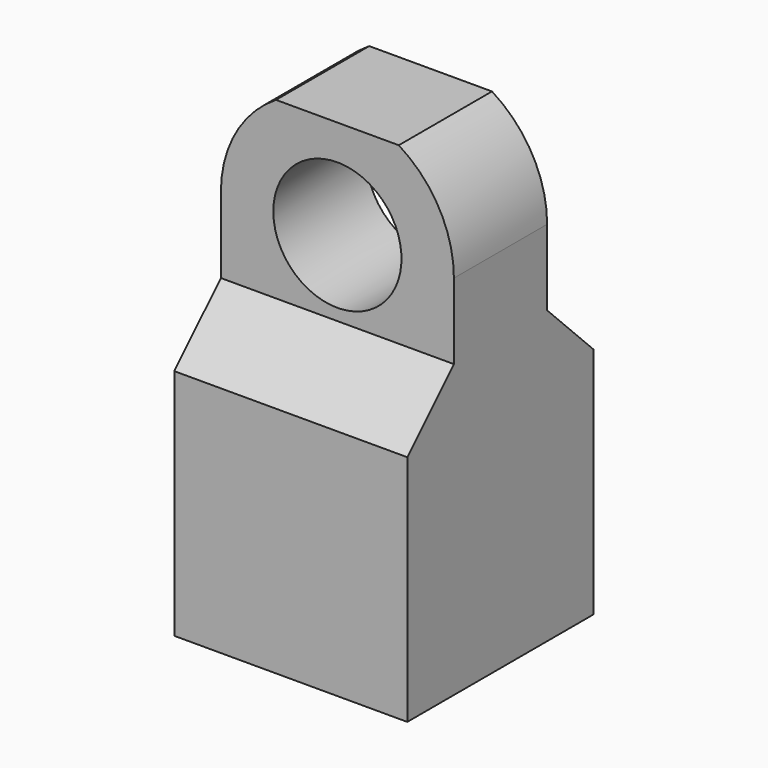
from build123d import *

# Parameters (mm, degrees)
F0_W      = 20
F0_H      = 20
F0_R      = 4
F1_DEPTH  = 25
F3_W      = 14
F3_H      = 5.8359876275
F4_DEPTH  = 17
F6_W      = 20
F6_H      = 10
F7_DEPTH  = 15
F10_DEPTH = 10
F9_R      = 5.5
F11_DEPTH = 10
F12_SIZE  = 4.99999


# Not quite as in the source:
# - a fillet or chamfer is up to 0.001 mm smaller than in the source, because OpenCascade refuses the exact size


with BuildPart() as f1:
    # F0 (on Top) → F1 (new body)
    with BuildSketch(Plane.XY):
        Rectangle(F0_W, F0_H)
        Circle(F0_R, mode=Mode.SUBTRACT)
    extrude(amount=F1_DEPTH)

    # F3 (on offset) → F4 (cut)
    with BuildSketch(Plane(origin=(0, 10, 0), x_dir=(-1, 0, 0), z_dir=(0, 1, 0))):
        with Locations((0, 12.9179938138)):
            Rectangle(F3_W, F3_H)
    extrude(amount=-F4_DEPTH, mode=Mode.SUBTRACT)

    # F6 (on offset) → F7 (join)
    with BuildSketch(Plane.XY.offset(25)):
        Rectangle(F6_W, F6_H)
    extrude(amount=F7_DEPTH)

    # F9 (on offset) → F10 (cut)
    with BuildSketch(Plane(origin=(0, 5, 0), x_dir=(-1, 0, 0), z_dir=(0, 1, 0))):
        with BuildLine():
            Line((-5.2678268764, 40), (-10, 40))
            Line((-10, 40), (-10, 31.5))
            ThreePointArc((-10, 31.5), (-8.7372269275, 36.3642435813), (-5.2678268764, 40))
        make_face()
        with BuildLine():
            Line((10, 40), (5.2678268764, 40))
            ThreePointArc((5.2678268764, 40), (8.7372269275, 36.3642435813), (10, 31.5))
            Line((10, 31.5), (10, 40))
        make_face()
    extrude(amount=-F10_DEPTH, mode=Mode.SUBTRACT)

    # F9 (on offset) → F11 (cut)
    with BuildSketch(Plane(origin=(0, 5, 0), x_dir=(-1, 0, 0), z_dir=(0, 1, 0))):
        with Locations((0, 31.5)):
            Circle(F9_R)
    extrude(amount=-F11_DEPTH, mode=Mode.SUBTRACT)

    # F12 (size 5 in the source; OpenCascade refuses exactly that, so slightly less here)
    f12_edges = [f1.edges().sort_by_distance(p)[0] for p in [
        (0, -10, 25),
        (0, 10, 25),
    ]]
    chamfer(f12_edges, length=F12_SIZE)


solid = f1.part
